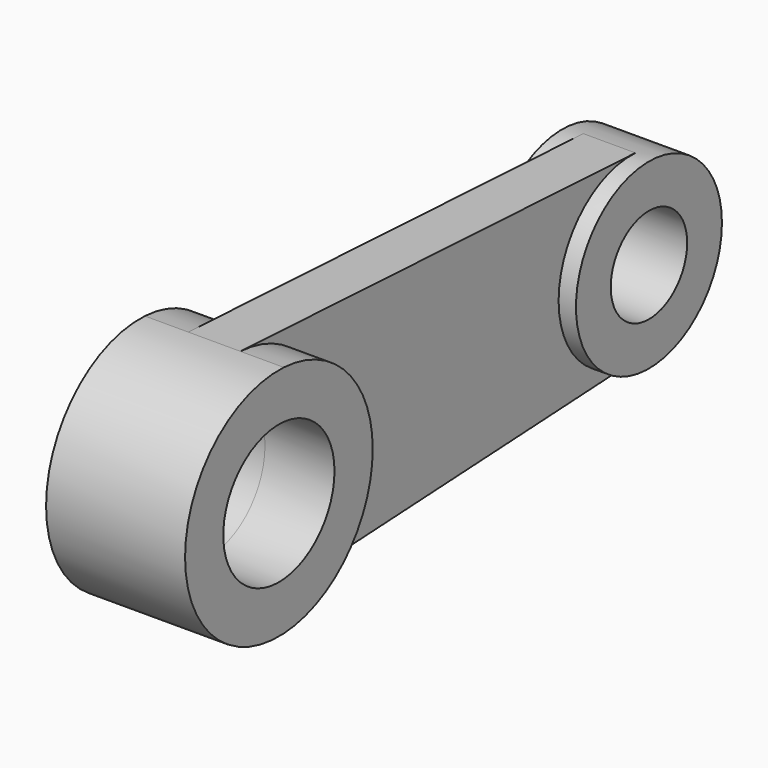
from build123d import *

# Parameters (mm, degrees)
F1_DEPTH = 9.525
F0_R     = 25.4
F2_DEPTH = 25.4
F0_R_2   = 17.4625
F3_DEPTH = 15.875


with BuildPart() as f1:
    # F0 (on Right) → F1 (new body, symmetric)
    with BuildSketch(Plane.YZ):
        with BuildLine():
            ThreePointArc((-35.9234930565, 42.803092487), (-7.0836883387, 29.4999956791), (4.6830858909, 0))
            ThreePointArc((4.6830858909, 0), (-7.0836883387, -29.4999956791), (-35.9234930565, -42.803092487))
            Line((-35.9234930565, -42.803092487), (144.5501911541, -33.2912941566))
            ThreePointArc((144.5501911541, -33.2912941566), (109.4580858909, 0), (144.5501911541, 33.2912941566))
            Line((144.5501911541, 33.2912941566), (-35.9234930565, 42.803092487))
        make_face()
    extrude(amount=F1_DEPTH, both=True)

    # F0 (on Right) → F2 (join, symmetric)
    with BuildSketch(Plane.YZ):
        with BuildLine():
            ThreePointArc((-35.9234930565, -42.803092487), (-7.0836883387, -29.4999956791), (4.6830858909, 0))
            ThreePointArc((4.6830858909, 0), (-7.0836883387, 29.4999956791), (-35.9234930565, 42.803092487))
            ThreePointArc((-35.9234930565, 42.803092487), (-81.0419141091, 0), (-35.9234930565, -42.803092487))
        make_face()
        with Locations((-38.1794141091, 0)):
            Circle(F0_R, mode=Mode.SUBTRACT)
    extrude(amount=F2_DEPTH, both=True)

    # F0 (on Right) → F3 (join, symmetric)
    with BuildSketch(Plane.YZ):
        with BuildLine():
            ThreePointArc((176.1330858909, 0), (166.981150379, 22.9444410837), (144.5501911541, 33.2912941566))
            ThreePointArc((144.5501911541, 33.2912941566), (109.4580858909, 0), (144.5501911541, -33.2912941566))
            ThreePointArc((144.5501911541, -33.2912941566), (166.981150379, -22.9444410837), (176.1330858909, 0))
        make_face()
        with Locations((142.7955858909, 0)):
            Circle(F0_R_2, mode=Mode.SUBTRACT)
    extrude(amount=F3_DEPTH, both=True)


solid = f1.part
